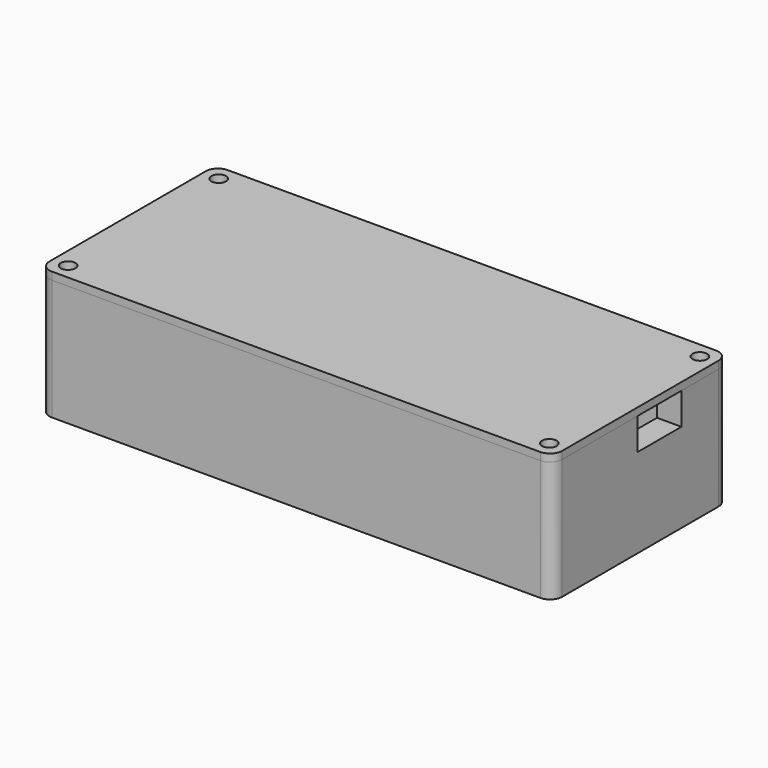
from build123d import *

# Parameters (mm, degrees)
F1_DEPTH = 19.558
F0_R     = 1.524
F2_DEPTH = 5.588
F3_R     = 1.524
F4_DEPTH = 12.7
F5_W     = 5.08
F5_H     = 11.43
F6_DEPTH = 6.604
F7_DEPTH = 4.318
F8_R     = 1.524
F9_DEPTH = 1.5875


# Not quite as in the source:
# - a length typed as a fraction of an inch, garbled in the dataset ("3 / 203.2 mm" for 3/8 in), is restored


with BuildPart() as f1:
    # F0 (on Top) → F1 (new body)
    with BuildSketch(Plane.XY):
        with BuildLine():
            Line((99.06, 40.64), (-2.54, 40.64))
            ThreePointArc((-2.54, 40.64), (-4.3360512242, 39.8960512242), (-5.08, 38.1))
            Line((-5.08, 38.1), (-5.08, -2.54))
            ThreePointArc((-5.08, -2.54), (-4.3360512242, -4.3360512242), (-2.54, -5.08))
            Line((-2.54, -5.08), (99.06, -5.08))
            ThreePointArc((99.06, -5.08), (100.8560512242, -4.3360512242), (101.6, -2.54))
            Line((101.6, -2.54), (101.6, 38.1))
            ThreePointArc((101.6, 38.1), (100.8560512242, 39.8960512242), (99.06, 40.64))
        make_face()
        with BuildLine():
            Line((93.98, 0), (2.54, 0))
            ThreePointArc((2.54, 0), (0.7439487758, 0.7439487758), (0, 2.54))
            Line((0, 2.54), (0, 33.02))
            ThreePointArc((0, 33.02), (0.7439487758, 34.8160512242), (2.54, 35.56))
            Line((2.54, 35.56), (93.98, 35.56))
            ThreePointArc((93.98, 35.56), (95.7760512242, 34.8160512242), (96.52, 33.02))
            Line((96.52, 33.02), (96.52, 2.54))
            ThreePointArc((96.52, 2.54), (95.7760512242, 0.7439487758), (93.98, 0))
        make_face(mode=Mode.SUBTRACT)
    extrude(amount=F1_DEPTH)

    # F0 (on Top) → F2 (join)
    with BuildSketch(Plane.XY):
        with BuildLine():
            Line((99.06, 40.64), (-2.54, 40.64))
            ThreePointArc((-2.54, 40.64), (-4.3360512242, 39.8960512242), (-5.08, 38.1))
            Line((-5.08, 38.1), (-5.08, -2.54))
            ThreePointArc((-5.08, -2.54), (-4.3360512242, -4.3360512242), (-2.54, -5.08))
            Line((-2.54, -5.08), (99.06, -5.08))
            ThreePointArc((99.06, -5.08), (100.8560512242, -4.3360512242), (101.6, -2.54))
            Line((101.6, -2.54), (101.6, 38.1))
            ThreePointArc((101.6, 38.1), (100.8560512242, 39.8960512242), (99.06, 40.64))
        make_face()
        with BuildLine():
            Line((93.98, 0), (2.54, 0))
            ThreePointArc((2.54, 0), (0.7439487758, 0.7439487758), (0, 2.54))
            Line((0, 2.54), (0, 33.02))
            ThreePointArc((0, 33.02), (0.7439487758, 34.8160512242), (2.54, 35.56))
            Line((2.54, 35.56), (93.98, 35.56))
            ThreePointArc((93.98, 35.56), (95.7760512242, 34.8160512242), (96.52, 33.02))
            Line((96.52, 33.02), (96.52, 2.54))
            ThreePointArc((96.52, 2.54), (95.7760512242, 0.7439487758), (93.98, 0))
        make_face(mode=Mode.SUBTRACT)
        with BuildLine():
            ThreePointArc((0, 2.54), (0.7439487758, 0.7439487758), (2.54, 0))
            Line((2.54, 0), (93.98, 0))
            ThreePointArc((93.98, 0), (95.7760512242, 0.7439487758), (96.52, 2.54))
            Line((96.52, 2.54), (96.52, 33.02))
            ThreePointArc((96.52, 33.02), (95.7760512242, 34.8160512242), (93.98, 35.56))
            Line((93.98, 35.56), (2.54, 35.56))
            ThreePointArc((2.54, 35.56), (0.7439487758, 34.8160512242), (0, 33.02))
            Line((0, 33.02), (0, 2.54))
        make_face()
        with Locations((4.699, 17.78)):
            Circle(F0_R, mode=Mode.SUBTRACT)
        with Locations((78.359, 17.78)):
            Circle(F0_R, mode=Mode.SUBTRACT)
        with Locations((78.359, 17.78)):
            Circle(F0_R)
        with Locations((4.699, 17.78)):
            Circle(F0_R)
    extrude(amount=-F2_DEPTH)

    # F3 (on face) → F4 (cut)
    with BuildSketch(Plane.XY.offset(19.558)):
        with Locations((-1.7960512242, -1.7960512242)):
            Circle(F3_R)
        with Locations((-1.7960512242, 37.3560512242)):
            Circle(F3_R)
        with Locations((98.3160512242, 37.3560512242)):
            Circle(F3_R)
        with Locations((98.3160512242, -1.7960512242)):
            Circle(F3_R)
    extrude(amount=-F4_DEPTH, mode=Mode.SUBTRACT)

    # F5 (on face) → F6 (cut)
    with BuildSketch(Plane.XY.offset(19.558)):
        with Locations((99.06, 22.733)):
            Rectangle(F5_W, F5_H)
    extrude(amount=-F6_DEPTH, mode=Mode.SUBTRACT)

    # F0 (on Top) → F7 (cut)
    with BuildSketch(Plane.XY):
        with Locations((4.699, 17.78)):
            Circle(F0_R)
        with Locations((78.359, 17.78)):
            Circle(F0_R)
    extrude(amount=-F7_DEPTH, mode=Mode.SUBTRACT)


with BuildPart() as f9:
    # F8 (on face) → F9 (new body)
    with BuildSketch(Plane.XY.offset(19.558)):
        with BuildLine():
            Line((99.06, 40.64), (-2.54, 40.64))
            ThreePointArc((-2.54, 40.64), (-4.3360512242, 39.8960512242), (-5.08, 38.1))
            Line((-5.08, 38.1), (-5.08, -2.54))
            ThreePointArc((-5.08, -2.54), (-4.3360512242, -4.3360512242), (-2.54, -5.08))
            Line((-2.54, -5.08), (99.06, -5.08))
            ThreePointArc((99.06, -5.08), (100.8560512242, -4.3360512242), (101.6, -2.54))
            Line((101.6, -2.54), (101.6, 38.1))
            ThreePointArc((101.6, 38.1), (100.8560512242, 39.8960512242), (99.06, 40.64))
        make_face()
        with Locations((-1.7960512242, -1.7960512242)):
            Circle(F8_R, mode=Mode.SUBTRACT)
        with Locations((98.3160512242, -1.7960512242)):
            Circle(F8_R, mode=Mode.SUBTRACT)
        with Locations((-1.7960512242, 37.3560512242)):
            Circle(F8_R, mode=Mode.SUBTRACT)
        with Locations((98.3160512242, 37.3560512242)):
            Circle(F8_R, mode=Mode.SUBTRACT)
    extrude(amount=F9_DEPTH)


solid = Compound([f1.part, f9.part])
